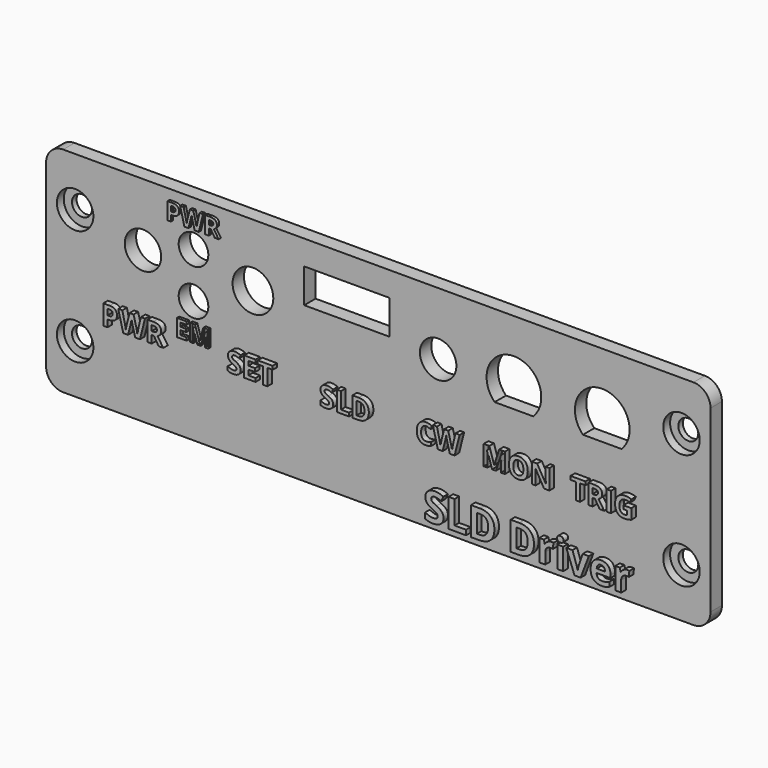
from build123d import *

# Parameters (mm, degrees)
F0_R          = 1.75
F1_DEPTH      = 2.5
F2_R          = 3.2
F3_DEPTH      = 1.5
F4_W          = 2.5
F4_H          = 6
F5_DEPTH      = 1.25
F6_R          = 3.575
F6_R_2        = 3.2
F6_W          = 15
F6_H          = 6
F6_R_3        = 2.6
F7_DEPTH      = 2.501
F8_TEXT_SIZE  = 4.8611111111
F9_DEPTH      = 1
F10_TEXT_SIZE = 6.9444444444
F11_DEPTH     = 1
F12_TEXT_SIZE = 4.1666666667
F13_DEPTH     = 0.5


# Not quite as in the source:
# - Text() gives the source's letters only with a copy of the font that has no kerning and outlines rounded to 1/6400 em; it was checked with that copy


with BuildPart() as f1:
    # F0 (on Front) → F1 (new body)
    with BuildSketch(Plane.XZ):
        with BuildLine():
            Line((55.3, 18.75), (-55.3, 18.75))
            ThreePointArc((-55.3, 18.75), (-57.4213203436, 17.8713203436), (-58.3, 15.75))
            Line((-58.3, 15.75), (-58.3, -15.75))
            ThreePointArc((-58.3, -15.75), (-57.4213203436, -17.8713203436), (-55.3, -18.75))
            Line((-55.3, -18.75), (55.3, -18.75))
            ThreePointArc((55.3, -18.75), (57.4213203436, -17.8713203436), (58.3, -15.75))
            Line((58.3, -15.75), (58.3, 15.75))
            ThreePointArc((58.3, 15.75), (57.4213203436, 17.8713203436), (55.3, 18.75))
        make_face()
        with Locations((-53.2, -10.15)):
            Circle(F0_R, mode=Mode.SUBTRACT)
        with Locations((53.2, -10.15)):
            Circle(F0_R, mode=Mode.SUBTRACT)
        with Locations((-53.2, 10.15)):
            Circle(F0_R, mode=Mode.SUBTRACT)
        with Locations((53.2, 10.15)):
            Circle(F0_R, mode=Mode.SUBTRACT)
    extrude(amount=F1_DEPTH)

    # F2 (on face) → F3 (cut)
    with BuildSketch(Plane.XZ.offset(2.5)):
        with Locations((-53.2, 10.15)):
            Circle(F2_R)
        with Locations((53.2, 10.15)):
            Circle(F2_R)
        with Locations((-53.2, -10.15)):
            Circle(F2_R)
        with Locations((53.2, -10.15)):
            Circle(F2_R)
    extrude(amount=-F3_DEPTH, mode=Mode.SUBTRACT)

    # F4 (on face) → F5 (cut)
    with BuildSketch(Plane(origin=(0, 0, 0), x_dir=(-1, 0, 0), z_dir=(0, 1, 0))):
        with Locations((57.05, 0)):
            Rectangle(F4_W, F4_H)
    extrude(amount=-F5_DEPTH, mode=Mode.SUBTRACT)

    # F6 (on face) → F7 (cut, through all)
    with BuildSketch(Plane.XZ.offset(2.5)):
        with BuildLine():
            Line((35.9117851308, 4.35), (42.6882148692, 4.35))
            ThreePointArc((42.6882148692, 4.35), (39.3, 12.55), (35.9117851308, 4.35))
        make_face()
        with Locations((-22, 7.75)):
            Circle(F6_R)
        with Locations((10.5, 7.75)):
            Circle(F6_R_2)
        with Locations((-5.5, 11.45)):
            Rectangle(F6_W, F6_H)
        with BuildLine():
            Line((20.4117851308, 4.35), (27.1882148692, 4.35))
            ThreePointArc((27.1882148692, 4.35), (23.8, 12.55), (20.4117851308, 4.35))
        make_face()
        with Locations((-41.3, 7.75)):
            Circle(F6_R_2)
        with Locations((-32.4288010597, 10.75)):
            Circle(F6_R_3)
        with Locations((-32.4288010597, 2.75)):
            Circle(F6_R_3)
    extrude(amount=-F7_DEPTH, mode=Mode.SUBTRACT)

    # F8 (on face) → F9 (join)
    with BuildSketch(Plane.XZ.offset(2.5)):
        with Locations((-47.8966750297, -5.5213214364)):
            Text('PWR', F8_TEXT_SIZE, font='Open Sans', font_style=FontStyle.BOLD, text_align=(TextAlign.LEFT, TextAlign.BOTTOM))
        with Locations((-25.8521041557, -5.5213214364)):
            Text('SET', F8_TEXT_SIZE, font='Open Sans', font_style=FontStyle.BOLD, text_align=(TextAlign.LEFT, TextAlign.BOTTOM))
        with Locations((-9.6049122512, -5.5213214364)):
            Text('SLD', F8_TEXT_SIZE, font='Open Sans', font_style=FontStyle.BOLD, text_align=(TextAlign.LEFT, TextAlign.BOTTOM))
        with Locations((7.270953618, -5.5213214364)):
            Text('CW   MON', F8_TEXT_SIZE, font='Open Sans', font_style=FontStyle.BOLD, text_align=(TextAlign.LEFT, TextAlign.BOTTOM))
        with Locations((34.4274640083, -5.5213214364)):
            Text('TRIG', F8_TEXT_SIZE, font='Open Sans', font_style=FontStyle.BOLD, text_align=(TextAlign.LEFT, TextAlign.BOTTOM))
    extrude(amount=F9_DEPTH)

    # F10 (on face) → F11 (join)
    with BuildSketch(Plane.XZ.offset(2.5)):
        with Locations((8.6862881064, -17.1977844553)):
            Text('SLD Driver', F10_TEXT_SIZE, font='Open Sans', font_style=FontStyle.BOLD, text_align=(TextAlign.LEFT, TextAlign.BOTTOM))
    extrude(amount=F11_DEPTH)

    # F12 (on face) → F13 (join)
    with BuildSketch(Plane.XZ.offset(2.5)):
        with Locations((-36.9962763943, 14.0866324853)):
            Text('PWR', F12_TEXT_SIZE, font='Open Sans', font_style=FontStyle.BOLD, text_align=(TextAlign.LEFT, TextAlign.BOTTOM))
        with Locations((-35.3191255741, -3.4102049416)):
            Text('EM', F12_TEXT_SIZE, font='Open Sans', font_style=FontStyle.BOLD, text_align=(TextAlign.LEFT, TextAlign.BOTTOM))
    extrude(amount=F13_DEPTH)


solid = f1.part
